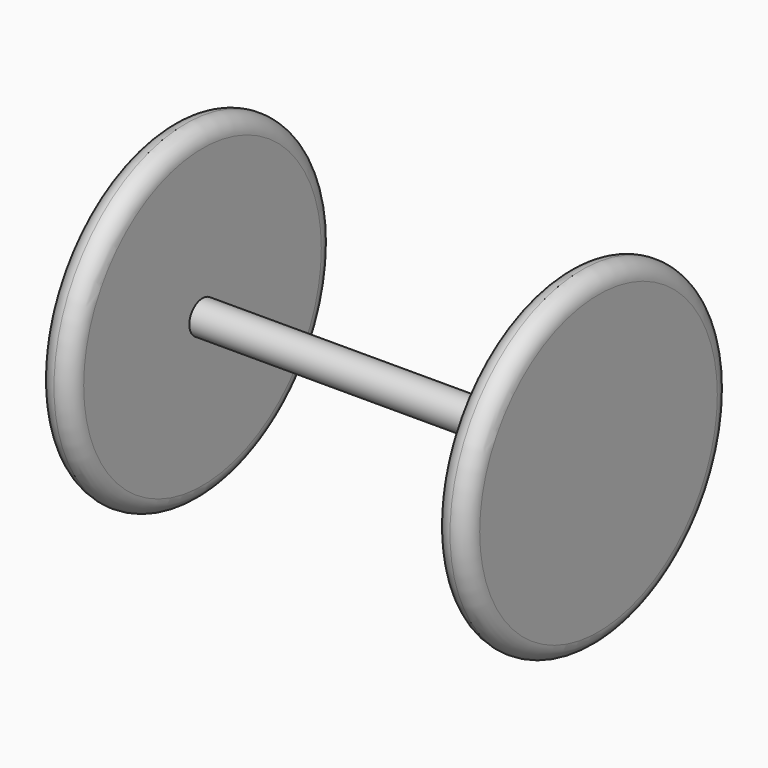
from build123d import *

# Parameters (mm, degrees)
F0_R     = 10
F1_DEPTH = 2
F2_R     = 1
F3_DEPTH = 22
F4_R     = 10
F5_DEPTH = 2
F6_R     = 0.99999


# Not quite as in the source:
# - a fillet or chamfer is up to 0.001 mm smaller than in the source, because OpenCascade refuses the exact size


with BuildPart() as f1:
    # F0 (on Right) → F1 (new body)
    with BuildSketch(Plane.YZ):
        with Locations((55.1835894585, 16.7251080275)):
            Circle(F0_R)
    extrude(amount=F1_DEPTH)

    # F2 (on face) → F3 (join)
    with BuildSketch(Plane.YZ.offset(2)):
        with Locations((55.1835894585, 16.7251080275)):
            Circle(F2_R)
    extrude(amount=F3_DEPTH)

    # F4 (on face) → F5 (join)
    with BuildSketch(Plane.YZ.offset(24)):
        with Locations((55.1835894585, 16.7251080275)):
            Circle(F4_R)
    extrude(amount=F5_DEPTH)

    # F6 (radius 1 in the source; OpenCascade refuses exactly that, so slightly less here)
    f6_edges = [f1.edges().sort_by_distance(p)[0] for p in [
        (2, 45.183589, 16.725108),
        (0, 45.183589, 16.725108),
        (26, 45.183589, 16.725108),
        (24, 45.183589, 16.725108),
    ]]
    fillet(f6_edges, radius=F6_R)


solid = f1.part
